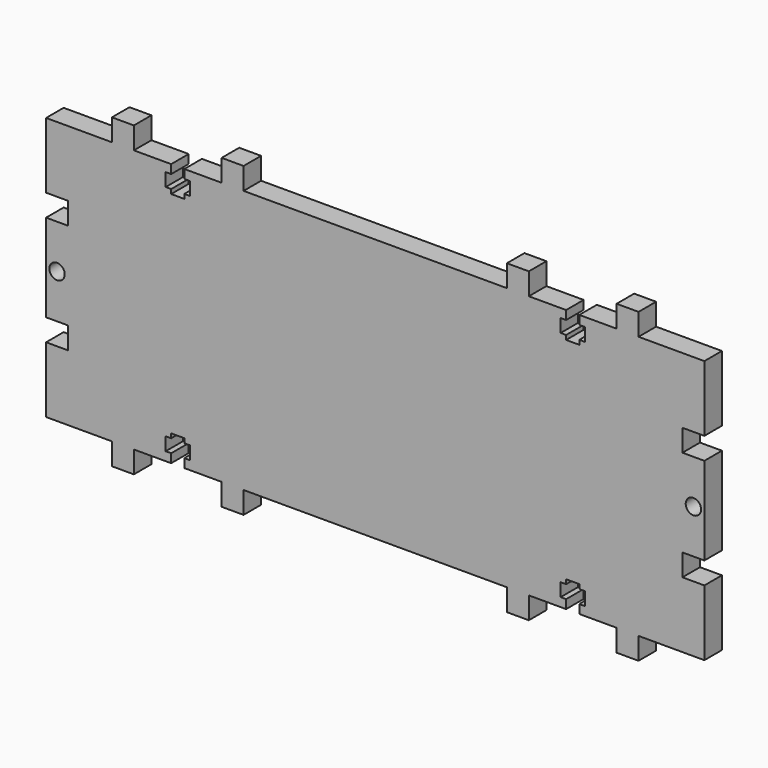
from build123d import *

# Parameters (mm, degrees)
F0_W     = 150
F0_H     = 5
F1_DEPTH = 60
F2_W     = 5
F2_H     = 5
F3_DEPTH = 5
F4_R     = 1.75
F4_W     = 5
F4_H     = 5
F5_DEPTH = 5


with BuildPart() as f1:
    # F0 (on Top) → F1 (new body)
    with BuildSketch(Plane.XY):
        with Locations((75, 2.5)):
            Rectangle(F0_W, F0_H)
    extrude(amount=F1_DEPTH)

    # F2 (on face) → F3 (join, through all)
    with BuildSketch(Plane.XZ):
        with Locations((17.5, -2.5)):
            Rectangle(F2_W, F2_H)
        with Locations((42.5, -2.5)):
            Rectangle(F2_W, F2_H)
        with Locations((107.5, -2.5)):
            Rectangle(F2_W, F2_H)
        with Locations((132.5, -2.5)):
            Rectangle(F2_W, F2_H)
        with Locations((42.5, 62.5)):
            Rectangle(F2_W, F2_H)
        with Locations((17.5, 62.5)):
            Rectangle(F2_W, F2_H)
        with Locations((132.5, 62.5)):
            Rectangle(F2_W, F2_H)
        with Locations((107.5, 62.5)):
            Rectangle(F2_W, F2_H)
    extrude(amount=-F3_DEPTH)

    # F4 (on face) → F5 (cut, through all)
    with BuildSketch(Plane.XZ):
        Polygon((28.5, 2), (28.5, 0), (31.5, 0), (31.5, 2), (32.75, 2), (32.75, 5), (31.5, 5), (31.5, 6), (28.5, 6), (28.5, 5), (27.25, 5), (27.25, 2), align=None)
        Polygon((118.5, 6), (118.5, 5), (117.25, 5), (117.25, 2), (118.5, 2), (118.5, 0), (121.5, 0), (121.5, 2), (122.75, 2), (122.75, 5), (121.5, 5), (121.5, 6), align=None)
        Polygon((121.5, 55), (122.75, 55), (122.75, 58), (121.5, 58), (121.5, 60), (118.5, 60), (118.5, 58), (117.25, 58), (117.25, 55), (118.5, 55), (118.5, 54), (121.5, 54), align=None)
        Polygon((31.5, 54), (31.5, 55), (32.75, 55), (32.75, 58), (31.5, 58), (31.5, 60), (28.5, 60), (28.5, 58), (27.25, 58), (27.25, 55), (28.5, 55), (28.5, 54), align=None)
        with Locations((2.5, 30)):
            Circle(F4_R)
        with Locations((2.5, 42.5)):
            Rectangle(F4_W, F4_H)
        with Locations((2.5, 17.5)):
            Rectangle(F4_W, F4_H)
        with Locations((147.5, 42.5)):
            Rectangle(F4_W, F4_H)
        with Locations((147.5, 30)):
            Circle(F4_R)
        with Locations((147.5, 17.5)):
            Rectangle(F4_W, F4_H)
    extrude(amount=-F5_DEPTH, mode=Mode.SUBTRACT)


solid = f1.part
